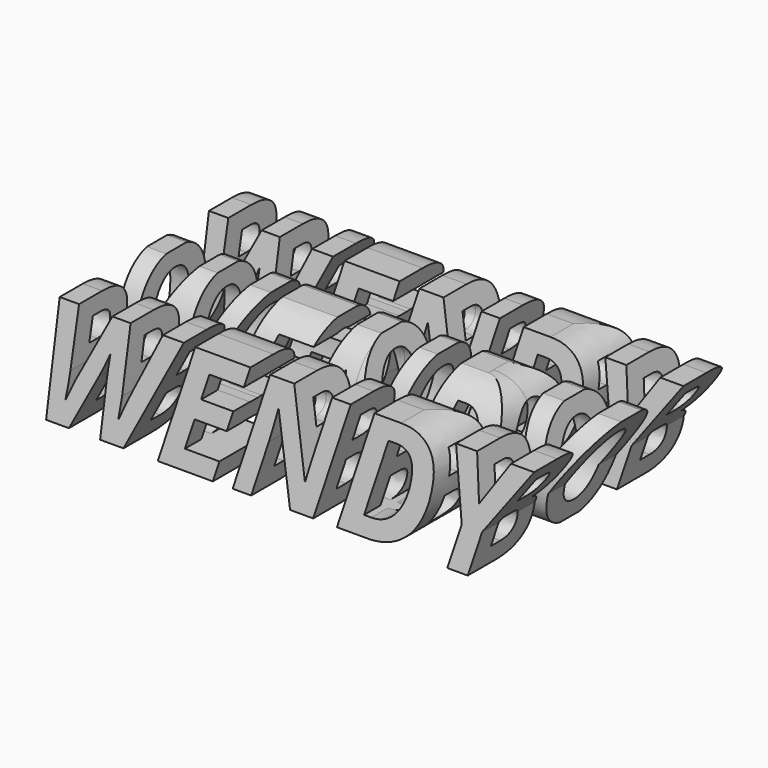
from build123d import *

# Parameters (mm, degrees)
F0_TEXT_SIZE  = 34.7222222222
F1_DEPTH      = 50
F1_DEPTH_BACK = 50
F2_TEXT_SIZE  = 34.7222222222
F3_DEPTH      = 75
F3_DEPTH_BACK = 75


# Not quite as in the source:
# - Text() gives the source's letters only with a copy of the font that has no kerning and outlines rounded to 1/6400 em; it was checked with that copy


with BuildPart() as f1:
    # F0 (on Front) → F1 (new body, two sides)
    with BuildSketch(Plane.XZ) as f1_sk:
        with Locations((-62.2965494792, 0)):
            Text('WENDY', F0_TEXT_SIZE, font='Open Sans', font_style=FontStyle.BOLDITALIC, text_align=(TextAlign.LEFT, TextAlign.BOTTOM))
    extrude(amount=F1_DEPTH)
    extrude(f1_sk.sketch, amount=-F1_DEPTH_BACK)


with BuildPart() as f3:
    # F2 (on Right) → F3 (new body, two sides)
    with BuildSketch(Plane.YZ) as f3_sk:
        with Locations((-35.1698133681, 0)):
            Text('BOB', F2_TEXT_SIZE, font='Open Sans', font_style=FontStyle.BOLDITALIC, text_align=(TextAlign.LEFT, TextAlign.BOTTOM))
    extrude(amount=F3_DEPTH)
    extrude(f3_sk.sketch, amount=-F3_DEPTH_BACK)

    # F4: intersect F1
    add(f1.part, mode=Mode.INTERSECT)


solid = f3.part
